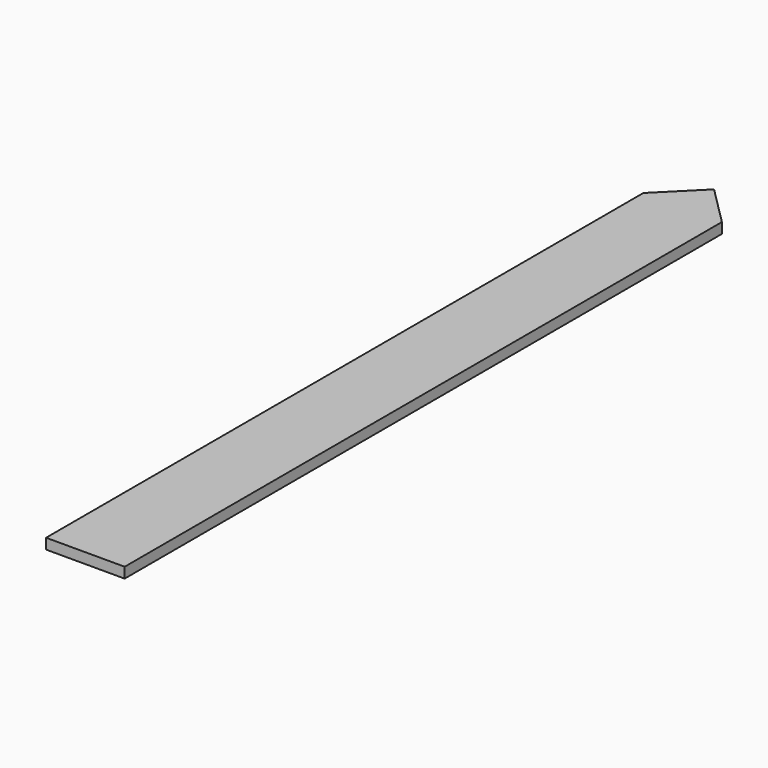
from build123d import *

# Parameters (mm, degrees)
F0_W     = 1.905
F0_H     = 19.05
F1_DEPTH = 0.254
F2_SIZE  = 0.9525
F3_SIZE  = 0.95249


# Not quite as in the source:
# - a fillet or chamfer is up to 0.001 mm smaller than in the source, because OpenCascade refuses the exact size


with BuildPart() as f1:
    # F0 (on Top) → F1 (new body)
    with BuildSketch(Plane.XY):
        with Locations((-0.9525, 9.525)):
            Rectangle(F0_W, F0_H)
    extrude(amount=F1_DEPTH)

    # F2
    f2_edges = [f1.edges().sort_by_distance(p)[0] for p in [
        (-1.905, 19.05, 0.127),
    ]]
    chamfer(f2_edges, length=F2_SIZE)

    # F3 (size 0.9525 in the source; OpenCascade refuses exactly that, so slightly less here)
    f3_edges = [f1.edges().sort_by_distance(p)[0] for p in [
        (0, 19.05, 0.127),
    ]]
    chamfer(f3_edges, length=F3_SIZE)


solid = f1.part
